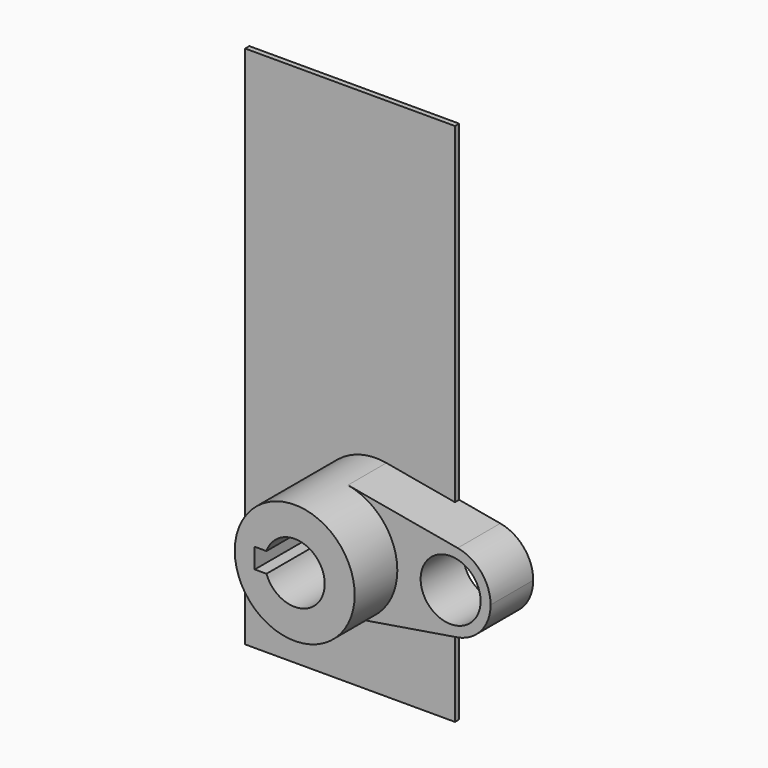
from build123d import *

# Parameters (mm, degrees)
F0_R     = 14.2875
F1_DEPTH = 25.4
F2_DEPTH = 50.8
F3_W     = 100
F3_H     = 250
F4_DEPTH = 2.5


# Not quite as in the source:
# - a feature of the source that left no trace in its solid (it failed there, or was rolled back) is left out


with BuildPart() as f1:
    # F0 (on Front) → F1 (new body)
    with BuildSketch(Plane.XZ):
        with BuildLine():
            ThreePointArc((11.2557435726, -26.2647836775), (23.8554343661, -15.7305078178), (28.575, 0))
            ThreePointArc((28.575, 0), (21.9160245563, 18.3362616868), (5.0426470588, 28.1265414802))
            ThreePointArc((5.0426470588, 28.1265414802), (-28.3903759644, -3.2430198275), (11.2557435726, -26.2647836775))
        make_face()
        with BuildLine():
            ThreePointArc((-13.4703841816, 4.7625), (0, 14.2875), (13.4703841816, 4.7625))
            Line((13.4703841816, 4.7625), (19.05, 4.7625))
            Line((19.05, 4.7625), (19.05, -4.7625))
            Line((19.05, -4.7625), (13.4703841816, -4.7625))
            ThreePointArc((13.4703841816, -4.7625), (0, -14.2875), (-13.4703841816, -4.7625))
            Line((-13.4703841816, -4.7625), (-19.05, -4.7625))
            Line((-19.05, -4.7625), (-19.05, 4.7625))
            Line((-19.05, 4.7625), (-13.4703841816, 4.7625))
        make_face(mode=Mode.SUBTRACT)
        with BuildLine():
            ThreePointArc((5.0426470588, 28.1265414802), (21.9160245563, 18.3362616868), (28.575, 0))
            ThreePointArc((28.575, 0), (23.8554343661, -15.7305078178), (11.2557435726, -26.2647836775))
            Line((11.2557435726, -26.2647836775), (57.0397573458, -18.8018552917))
            ThreePointArc((57.0397573458, -18.8018552917), (34.925595789, 0.1506625541), (57.3367647059, 18.7510276535))
            Line((57.3367647059, 18.7510276535), (5.0426470588, 28.1265414802))
        make_face()
        with BuildLine():
            ThreePointArc((73.025, 0), (68.5856830375, 12.2241744579), (57.3367647059, 18.7510276535))
            ThreePointArc((57.3367647059, 18.7510276535), (34.925595789, 0.1506625541), (57.0397573458, -18.8018552917))
            ThreePointArc((57.0397573458, -18.8018552917), (68.4885475925, -12.3393450508), (73.025, 0))
        make_face()
        with Locations((53.975, 0)):
            Circle(F0_R, mode=Mode.SUBTRACT)
    extrude(amount=F1_DEPTH)

    # F0 (on Front) → F2 (join)
    with BuildSketch(Plane.XZ):
        with BuildLine():
            ThreePointArc((11.2557435726, -26.2647836775), (23.8554343661, -15.7305078178), (28.575, 0))
            ThreePointArc((28.575, 0), (21.9160245563, 18.3362616868), (5.0426470588, 28.1265414802))
            ThreePointArc((5.0426470588, 28.1265414802), (-28.3903759644, -3.2430198275), (11.2557435726, -26.2647836775))
        make_face()
        with BuildLine():
            ThreePointArc((-13.4703841816, 4.7625), (0, 14.2875), (13.4703841816, 4.7625))
            Line((13.4703841816, 4.7625), (19.05, 4.7625))
            Line((19.05, 4.7625), (19.05, -4.7625))
            Line((19.05, -4.7625), (13.4703841816, -4.7625))
            ThreePointArc((13.4703841816, -4.7625), (0, -14.2875), (-13.4703841816, -4.7625))
            Line((-13.4703841816, -4.7625), (-19.05, -4.7625))
            Line((-19.05, -4.7625), (-19.05, 4.7625))
            Line((-19.05, 4.7625), (-13.4703841816, 4.7625))
        make_face(mode=Mode.SUBTRACT)
        with BuildLine():
            ThreePointArc((13.4703841816, 4.7625), (14.081739421, 2.416044521), (14.2875, 0))
            ThreePointArc((14.2875, 0), (14.081739421, -2.416044521), (13.4703841816, -4.7625))
            Line((13.4703841816, -4.7625), (19.05, -4.7625))
            Line((19.05, -4.7625), (19.05, 4.7625))
            Line((19.05, 4.7625), (13.4703841816, 4.7625))
        make_face()
    extrude(amount=F2_DEPTH)


with BuildPart() as f4:
    # F3 (on Front) → F4 (new body)
    with BuildSketch(Plane.XZ):
        with Locations((-12.2774355114, 55.1020845771)):
            Rectangle(F3_W, F3_H)
    extrude(amount=F4_DEPTH)


solid = Compound([f1.part, f4.part])
